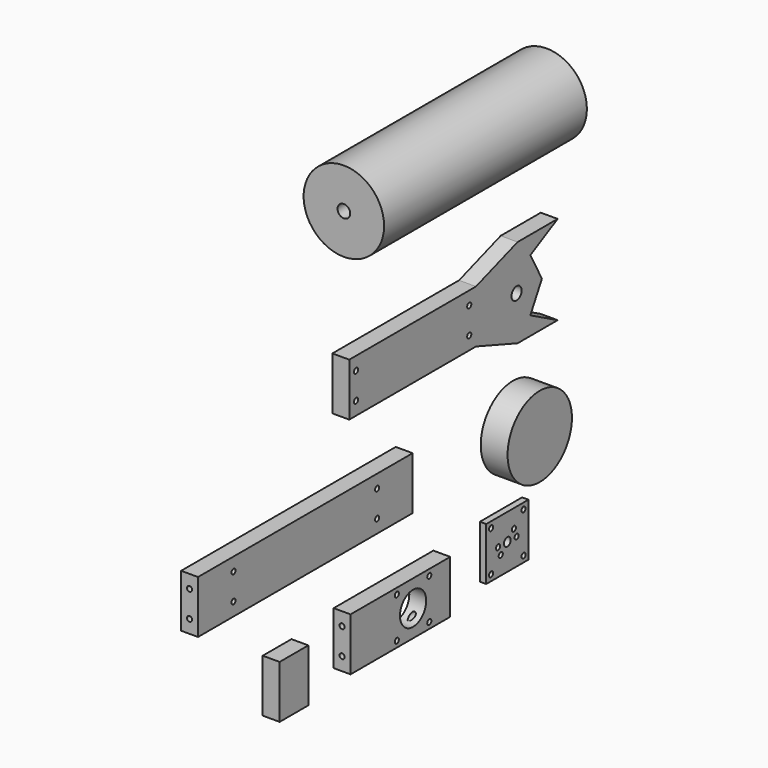
from build123d import *

# Parameters (mm, degrees)
F0_R      = 1.219
F0_R_2    = 3
F1_DEPTH  = 8
F2_W      = 127
F2_H      = 25
F2_R      = 1.219
F3_DEPTH  = 8
F4_R      = 19.05
F5_DEPTH  = 12.7
F6_W      = 17
F6_H      = 25
F8_DEPTH  = 8
F7_W      = 59
F7_H      = 25
F7_R      = 1.219
F7_R_2    = 7.75
F9_DEPTH  = 8
F10_R     = 19.05
F11_DEPTH = 120
F12_R     = 1.219
F13_DEPTH = 10
F14_R     = 1.219
F15_DEPTH = 10
F16_R     = 1.219
F17_DEPTH = 100
F18_W     = 25
F18_H     = 25
F18_R     = 1.219
F18_R_2   = 2
F19_DEPTH = 3
F20_R     = 3
F21_DEPTH = 25


# Not quite as in the source:
# - a feature names something its author has since deleted; it is built from what else it names


with BuildPart() as f1:
    # F0 (on Right) → F1 (new body)
    with BuildSketch(Plane.YZ):
        Polygon((72.5721682824, 11.3142699003), (-2.4278317176, 11.3142699003), (-2.4278317176, -13.6857300997), (72.5721682824, -13.6857300997), (97.2220564368, -22.3569506155), (120.9023296833, -22.3569506155), (104.7430932522, -13.778945595), (111.5817129612, -1.2896135449), (104.7430932522, 11.3036019504), (120.9023296833, 19.8494932056), (97.1770928144, 19.8494932056), align=None)
        with Locations((1.5721682824, -7.4357300997)):
            Circle(F0_R, mode=Mode.SUBTRACT)
        with Locations((68.5721682824, -7.4357300997)):
            Circle(F0_R, mode=Mode.SUBTRACT)
        with Locations((96.5817129612, -1.2896135449)):
            Circle(F0_R_2, mode=Mode.SUBTRACT)
        with Locations((1.5721682824, 5.0642699003)):
            Circle(F0_R, mode=Mode.SUBTRACT)
        with Locations((68.5721682824, 5.0642699003)):
            Circle(F0_R, mode=Mode.SUBTRACT)
    extrude(amount=F1_DEPTH)


with BuildPart() as f3:
    # F2 (on Right) → F3 (new body)
    with BuildSketch(Plane.YZ):
        with Locations((-28.4287979603, -55.3949028254)):
            Rectangle(F2_W, F2_H)
        with Locations((-70.9287979603, -61.6449028254)):
            Circle(F2_R, mode=Mode.SUBTRACT)
        with Locations((14.0712020397, -61.6449028254)):
            Circle(F2_R, mode=Mode.SUBTRACT)
        with Locations((-70.9287979603, -49.1449028254)):
            Circle(F2_R, mode=Mode.SUBTRACT)
        with Locations((14.0712020397, -49.1449028254)):
            Circle(F2_R, mode=Mode.SUBTRACT)
    extrude(amount=F3_DEPTH)

    # F12 (on face) → F13 (cut)
    with BuildSketch(Plane(origin=(0, 35.0712020397, 0), x_dir=(-1, 0, 0), z_dir=(0, 1, 0))):
        with Locations((-4, -49.1449028254)):
            Circle(F12_R)
        with Locations((-4, -61.6449028254)):
            Circle(F12_R)
    extrude(amount=-F13_DEPTH, mode=Mode.SUBTRACT)

    # F14 (on face) → F15 (cut)
    with BuildSketch(Plane.XZ.offset(91.9287979603)):
        with Locations((4, -49.1449028254)):
            Circle(F14_R)
        with Locations((4, -61.6449028254)):
            Circle(F14_R)
    extrude(amount=-F15_DEPTH, mode=Mode.SUBTRACT)


with BuildPart() as f5:
    # F4 (on Right) → F5 (new body)
    with BuildSketch(Plane.YZ):
        with Locations((104.4337153435, -62.5775009394)):
            Circle(F4_R)
    extrude(amount=F5_DEPTH)


with BuildPart() as f8:
    # F6 (on Right) → F8 (new body)
    with BuildSketch(Plane.YZ):
        with Locations((-35.131787325, -110.4173436761)):
            Rectangle(F6_W, F6_H)
    extrude(amount=F8_DEPTH)


with BuildPart() as f9:
    # F7 (on Right) → F9 (new body)
    with BuildSketch(Plane.YZ):
        with Locations((27.8338990211, -107.6586810813)):
            Rectangle(F7_W, F7_H)
        with Locations((25.7285605055, -117.2640195969)):
            Circle(F7_R, mode=Mode.SUBTRACT)
        with Locations((44.9392375368, -117.2640195969)):
            Circle(F7_R, mode=Mode.SUBTRACT)
        with Locations((35.3338990211, -107.6586810813)):
            Circle(F7_R_2, mode=Mode.SUBTRACT)
        with Locations((25.7285605055, -98.0533425656)):
            Circle(F7_R, mode=Mode.SUBTRACT)
        with Locations((44.9392375368, -98.0533425656)):
            Circle(F7_R, mode=Mode.SUBTRACT)
    extrude(amount=F9_DEPTH)

    # F16 (on face) → F17 (cut)
    with BuildSketch(Plane(origin=(0, 57.3338990211, 0), x_dir=(-1, 0, 0), z_dir=(0, 1, 0))):
        with Locations((-4, -101.4086810813)):
            Circle(F16_R)
        with Locations((-4, -113.9086810813)):
            Circle(F16_R)
    extrude(amount=-F17_DEPTH, mode=Mode.SUBTRACT)


with BuildPart() as f11:
    # F10 (on Front) → F11 (new body)
    with BuildSketch(Plane.XZ):
        with Locations((3.5049319267, 70.7618370652)):
            Circle(F10_R)
    extrude(amount=-F11_DEPTH)

    # F20 (on face) → F21 (cut)
    with BuildSketch(Plane.XZ):
        with Locations((3.5049319267, 70.7618370652)):
            Circle(F20_R)
    extrude(amount=-F21_DEPTH, mode=Mode.SUBTRACT)


with BuildPart() as f19:
    # F18 (on Right) → F19 (new body)
    with BuildSketch(Plane.YZ):
        with Locations((97.371138899, -106.8205982447)):
            Rectangle(F18_W, F18_H)
        with Locations((87.7661001213, -116.4256370224)):
            Circle(F18_R, mode=Mode.SUBTRACT)
        with Locations((93.4820516025, -110.7096855412)):
            Circle(F18_R, mode=Mode.SUBTRACT)
        with Locations((106.9761776768, -116.4256370224)):
            Circle(F18_R, mode=Mode.SUBTRACT)
        with Locations((91.871138899, -106.8205982447)):
            Circle(F18_R, mode=Mode.SUBTRACT)
        with Locations((87.7661001213, -97.2155594669)):
            Circle(F18_R, mode=Mode.SUBTRACT)
        with Locations((97.371138899, -106.8205982447)):
            Circle(F18_R_2, mode=Mode.SUBTRACT)
        with Locations((102.871138899, -106.8205982447)):
            Circle(F18_R, mode=Mode.SUBTRACT)
        with Locations((101.2602261955, -102.9315109481)):
            Circle(F18_R, mode=Mode.SUBTRACT)
        with Locations((106.9761776768, -97.2155594669)):
            Circle(F18_R, mode=Mode.SUBTRACT)
    extrude(amount=F19_DEPTH)


solid = Compound([f1.part, f3.part, f5.part, f8.part, f9.part, f11.part, f19.part])
